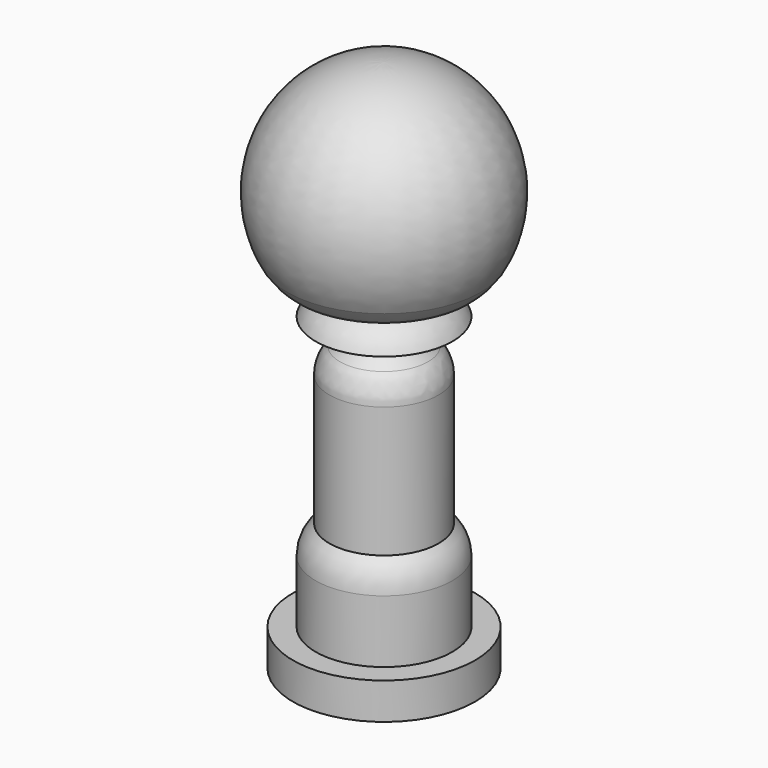
from build123d import *

# Parameters (mm, degrees)
F0_R      = 12.7
F1_DEPTH  = 5.08
F2_R      = 9.525
F3_DEPTH  = 12.7
F4_R      = 7.62
F5_DEPTH  = 25.4
F7_SIZE   = 5.08
F8_R      = 5.08
F9_R      = 9.525
F10_DEPTH = 3.81


# Not quite as in the source:
# - a fillet or chamfer that OpenCascade refuses, or shapes differently, is made with other operations: its cross-section is extruded or revolved along the edge and cut away or added


with BuildPart() as f1:
    # F0 (on Top) → F1 (new body)
    with BuildSketch(Plane.XY):
        Circle(F0_R)
    extrude(amount=F1_DEPTH)

    # F2 (on face) → F3 (join)
    with BuildSketch(Plane.XY.offset(5.08)):
        Circle(F2_R)
    extrude(amount=F3_DEPTH)

    # F4 (on face) → F5 (join)
    with BuildSketch(Plane.XY.offset(17.78)):
        Circle(F4_R)
    extrude(amount=F5_DEPTH)

    # F6: fillet of radius 5.08 on 1 edges, made by hand

    # F6_s1 → F6_t2 (revolve, cut)
    with BuildSketch(Plane.XZ):
        with BuildLine():
            ThreePointArc((9.525, 13.814426271), (9.0240501198, 16.0141307966), (7.62, 17.78))
            Line((7.62, 17.78), (9.525, 17.78))
            Line((9.525, 17.78), (9.525, 13.814426271))
        make_face()
    revolve(axis=Axis((0, 0, 17.78), (0, 0, 1)), mode=Mode.SUBTRACT)

    # F7
    f7_edges = [f1.edges().sort_by_distance(p)[0] for p in [
        (-7.62, 0, 43.18),
    ]]
    chamfer(f7_edges, length=F7_SIZE)

    # F8
    f8_edges = [f1.edges().sort_by_distance(p)[0] for p in [
        (-7.62, 0, 38.1),
    ]]
    fillet(f8_edges, radius=F8_R)

    # F9 (on face) → F10 (join)
    with BuildSketch(Plane.XY.offset(43.18)):
        Circle(F9_R)
    extrude(amount=F10_DEPTH)

    # F11: fillet of radius 6.1321024484 on 1 edges, made by hand

    # F11_s1 → F11_t2 (revolve, cut)
    with BuildSketch(Plane.XZ):
        with BuildLine():
            ThreePointArc((9.525, 43.18), (7.2674123234, 45.9491670665), (3.849568681, 46.99))
            Line((3.849568681, 46.99), (9.525, 46.99))
            Line((9.525, 46.99), (9.525, 43.18))
        make_face()
    revolve(axis=Axis((0, 0, 46.99), (0, 0, 1)), mode=Mode.SUBTRACT)


with BuildPart() as f13:
    # F12 (on Right) → F13 (revolve)
    with BuildSketch(Plane.YZ):
        with BuildLine():
            Line((0, 74.3997703671), (0, 47.5411827339))
            Line((0, 47.5411827339), (8.8249929249, 47.5411827339))
            add(Edge.make_bspline(
                [(13.5200609776, 50.5266902082), (12.9195581094, 49.6818747529), (11.726310154, 48.0196735533), (9.7842070151, 47.6986270543), (8.8249929249, 47.5411827339)],
                knots=[0, 0, 0, 0, 0.5066518371, 1, 1, 1, 1], degree=3))
            add(Edge.make_bspline(
                [(13.5200609776, 50.5266902082), (26.9612288802, 74.3997703671), (0, 74.3997703671)],
                knots=[1.0488861525, 1.0488861525, 1.0488861525, 3.1415926536, 3.1415926536, 3.1415926536], degree=2, weights=[1, 0.5007310075, 1]))
        make_face()
    revolve(axis=Axis((0, 0, 35.6023046188), (0, 0, -1)))


solid = Compound([f1.part, f13.part])
